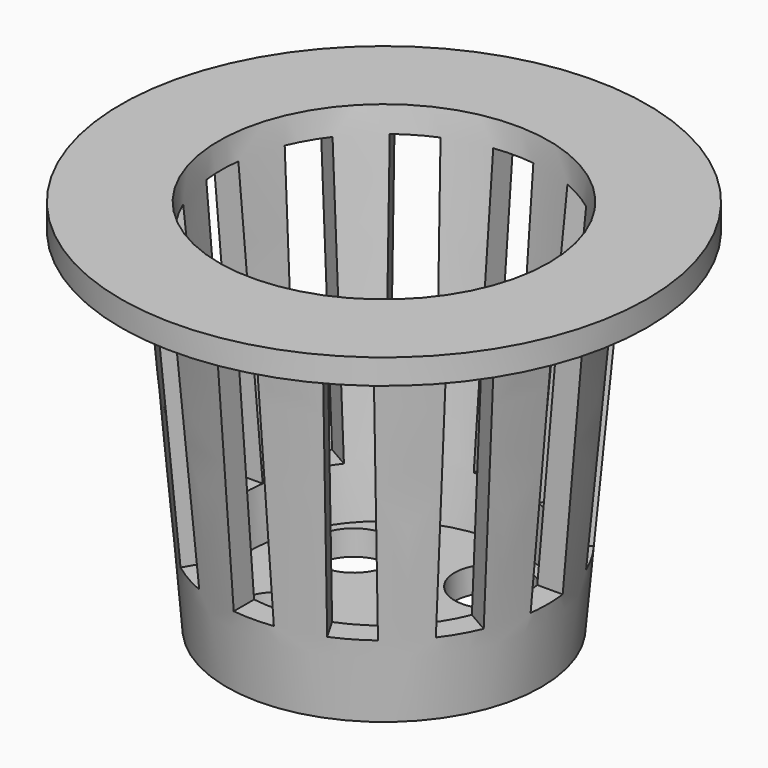
from build123d import *

# Parameters (mm, degrees)
F2_W            = 1.6
F2_H            = 11
F3_DEPTH        = 10.501
F3_COPIES_COUNT = 12
F4_R            = 1.5
F5_DEPTH        = 25


# Not quite as in the source:
# - a pattern or mirror of a feature is missing from the dataset's text; its kind, count and spacing are read off the source's solid


with BuildPart() as f1:
    # F0 (on Front) → F1 (revolve)
    with BuildSketch(Plane.XZ):
        Polygon((7.5, 14), (10.5, 14), (10.5, 15), (6.583668826, 15), (5.3588275366, 1), (0, 1), (0, 0), (6.2751587106, 0), align=None)
    revolve(axis=Axis((0, 0, 0.5), (0, 0, 1)))

    # F2 (on Right) → F3 (cut, through all)
    with BuildSketch(Plane.YZ):
        with Locations((0, 8.5)):
            Rectangle(F2_W, F2_H)
    f3 = extrude(amount=F3_DEPTH, mode=Mode.SUBTRACT)

    # F3_copies: F3 ×12 about axis
    f3_copies_axis = Axis((0, 0, 0), (0, 0, 1))
    for i in range(1, F3_COPIES_COUNT):
        add(f3.rotate(f3_copies_axis, i * 360 / F3_COPIES_COUNT), mode=Mode.SUBTRACT)

    # F4 (on face) → F5 (cut)
    with BuildSketch(Plane(origin=(0, 0, 0), x_dir=(1, 0, 0), z_dir=(0, 0, -1))):
        with Locations((-2.8413153179, -2.0437532298)):
            Circle(F4_R)
        with Locations((-2.0437532298, 2.8413153179)):
            Circle(F4_R)
        with Locations((2.8413153179, 2.0437532298)):
            Circle(F4_R)
        with Locations((2.0437532298, -2.8413153179)):
            Circle(F4_R)
    extrude(amount=-F5_DEPTH, mode=Mode.SUBTRACT)


solid = f1.part
